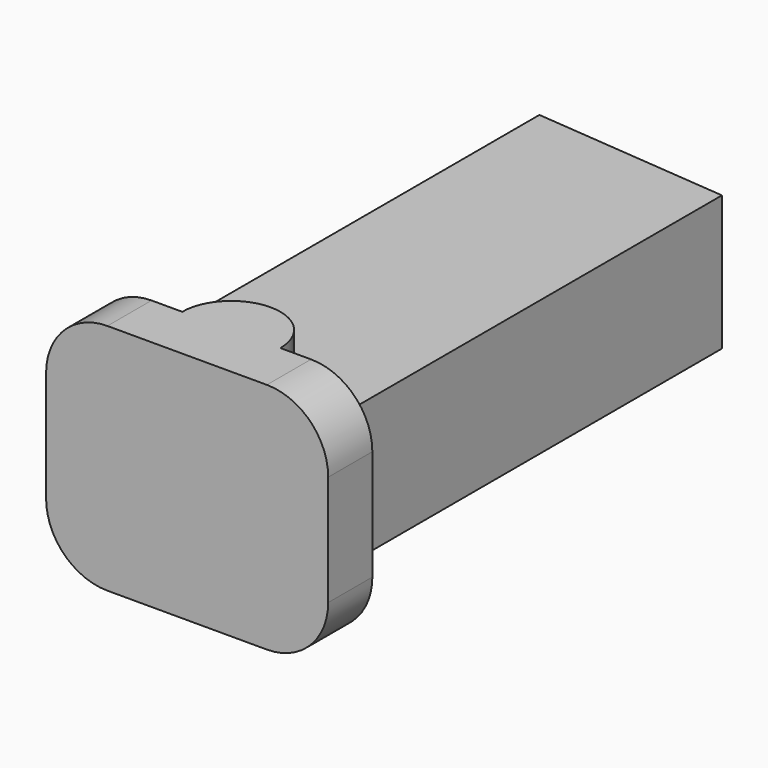
from build123d import *

# Parameters (mm, degrees)
F1_DEPTH = 5.5
F2_DEPTH = 9.5
F3_W     = 12
F3_H     = 7
F4_DEPTH = 44.1
F6_DEPTH = 4
F8_DEPTH = 4
F9_R     = 5
F10_R    = 5
F11_R    = 5
F12_R    = 5


# Not quite as in the source:
# - a feature names something its author has since deleted; it is built from what else it names


with BuildPart() as f1:
    # F0 (on Top) → F1 (new body, symmetric)
    with BuildSketch(Plane.XY):
        Polygon((41.8999169252, -11.2350502836), (25.8999169252, -9.8352316672), (25.8999169252, -51.2350502836), (41.8999169252, -51.2350502836), align=None)
    extrude(amount=F1_DEPTH, both=True)

    # F0 (on Top) → F2 (join, symmetric)
    with BuildSketch(Plane.XY):
        Polygon((41.8999169252, -51.2350502836), (25.8999169252, -51.2350502836), (22.3999169252, -51.2350502836), (22.3999169252, -55.7350502836), (45.3999169252, -55.7350502836), (45.3999169252, -51.2350502836), align=None)
    extrude(amount=F2_DEPTH, both=True)

    # F3 (on face) → F4 (cut)
    with BuildSketch(Plane(origin=(0, -51.2350502836, 0), x_dir=(-1, 0, 0), z_dir=(0, 1, 0))):
        with Locations((-33.8999169252, 0)):
            Rectangle(F3_W, F3_H)
    extrude(amount=F4_DEPTH, mode=Mode.SUBTRACT)

    # F5 (on face) → F6 (join)
    with BuildSketch(Plane.XY.offset(5.5)):
        with BuildLine():
            Line((29.8999169252, -51.2350502836), (37.8999169252, -51.2350502836))
            ThreePointArc((37.8999169252, -51.2350502836), (33.8999169252, -47.2350502836), (29.8999169252, -51.2350502836))
        make_face()
    extrude(amount=F6_DEPTH)

    # F7 (on face) → F8 (join)
    with BuildSketch(Plane(origin=(0, 0, -5.5), x_dir=(1, 0, 0), z_dir=(0, 0, -1))):
        with BuildLine():
            ThreePointArc((29.8999169252, 51.2350502836), (33.8999169252, 47.2350502836), (37.8999169252, 51.2350502836))
            Line((37.8999169252, 51.2350502836), (29.8999169252, 51.2350502836))
        make_face()
    extrude(amount=F8_DEPTH)

    # F9
    f9_edges = [f1.edges().sort_by_distance(p)[0] for p in [
        (22.399917, -53.48505, 9.5),
    ]]
    fillet(f9_edges, radius=F9_R)

    # F10
    f10_edges = [f1.edges().sort_by_distance(p)[0] for p in [
        (45.399917, -53.48505, 9.5),
    ]]
    fillet(f10_edges, radius=F10_R)

    # F11
    f11_edges = [f1.edges().sort_by_distance(p)[0] for p in [
        (45.399917, -53.48505, -9.5),
    ]]
    fillet(f11_edges, radius=F11_R)

    # F12
    f12_edges = [f1.edges().sort_by_distance(p)[0] for p in [
        (22.399917, -53.48505, -9.5),
    ]]
    fillet(f12_edges, radius=F12_R)


solid = f1.part
